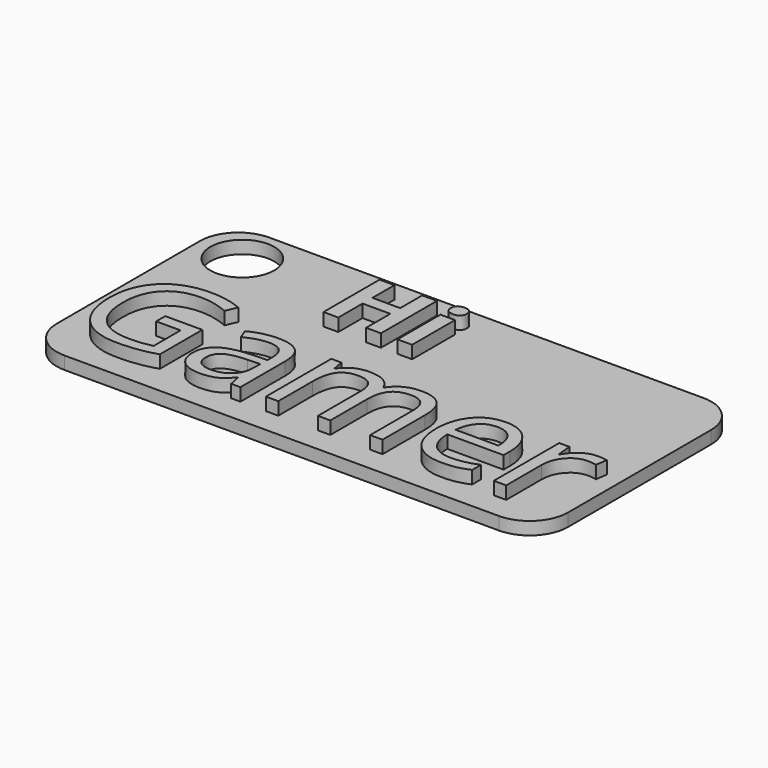
from build123d import *

# Parameters (mm, degrees)
F0_W         = 40
F0_H         = 20
F1_DEPTH     = 1
F2_R         = 3
F3_TEXT_SIZE = 11.9565226164
F4_DEPTH     = 1
F6_D         = 5
F6_DEPTH     = 50
F6_TIP       = 1.5021515476
F7_TEXT_SIZE = 7.6864228403
F8_DEPTH     = 1


# Not quite as in the source:
# - Text() gives the source's letters only with a copy of the font that has no kerning and outlines rounded to 1/6400 em; it was checked with that copy


with BuildPart() as f1:
    # F0 (on Top) → F1 (new body)
    with BuildSketch(Plane.XY):
        Rectangle(F0_W, F0_H)
    extrude(amount=F1_DEPTH)

    # F2
    f2_edges = [f1.edges().sort_by_distance(p)[0] for p in [
        (-20, 10, 0.5),
        (-20, -10, 0.5),
        (20, -10, 0.5),
        (20, 10, 0.5),
    ]]
    fillet(f2_edges, radius=F2_R)

    # F3 (on face) → F4 (join)
    with BuildSketch(Plane.XY.offset(1)):
        with Locations((-19.1739124712, -8.0593588063)):
            Text('Gamer', F3_TEXT_SIZE, font='Open Sans', text_align=(TextAlign.LEFT, TextAlign.BOTTOM))
    extrude(amount=F4_DEPTH)

    # F6
    with Locations(Plane.XY.offset(1)):
        with Locations((-16.5217090398, 6.7925113253)):
            Hole(F6_D / 2, depth=F6_DEPTH)
            with Locations((0, 0, -(F6_DEPTH + F6_TIP / 2))):  # 118° drill point
                Cone(0, F6_D / 2, F6_TIP, mode=Mode.SUBTRACT)

    # F7 (on face) → F8 (join)
    with BuildSketch(Plane.XY.offset(1)):
        with Locations((-7.7265226282, 2.8744291048)):
            Text('Hi', F7_TEXT_SIZE, font='Open Sans', font_style=FontStyle.BOLD, text_align=(TextAlign.LEFT, TextAlign.BOTTOM))
    extrude(amount=F8_DEPTH)


solid = f1.part
